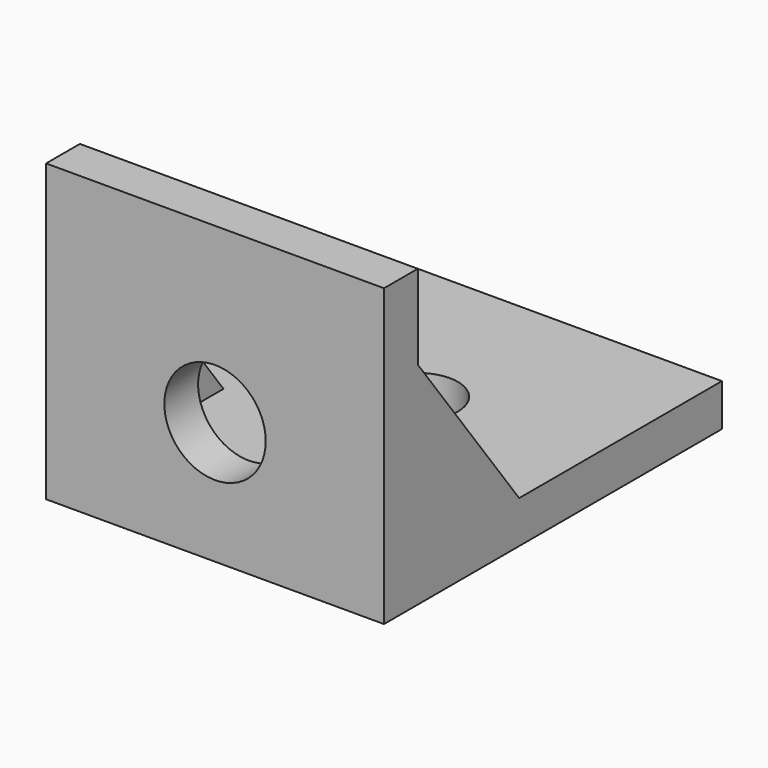
from build123d import *

# Parameters (mm, degrees)
F0_W       = 20
F0_H       = 25
F0_R       = 2.375
F1_DEPTH   = 2.5
F3_DEPTH   = 10
F4_SIZE2   = 7.49999
F4_SIZE    = 9.99999
F4_2_SIZE2 = 7.49999
F4_2_SIZE  = 9.99999
F5_DEPTH   = 5
F6_R       = 3
F7_DEPTH   = 2.5


# Not quite as in the source:
# - a fillet or chamfer is up to 0.001 mm smaller than in the source, because OpenCascade refuses the exact size


with BuildPart() as f1:
    # F0 (on Top) → F1 (new body)
    with BuildSketch(Plane.XY):
        with Locations((-35.0395915519, -25.5869545043)):
            Rectangle(F0_W, F0_H)
        with Locations((-35.0395915519, -23.0869545043)):
            Circle(F0_R, mode=Mode.SUBTRACT)
    extrude(amount=F1_DEPTH)

    # F2 (on face) → F3 (join)
    with BuildSketch(Plane.XY.offset(2.5)):
        Polygon((-42.5395915519, -28.0869545043), (-45.0395915519, -28.0869545043), (-45.0395915519, -38.0869545043), (-25.0395915519, -38.0869545043), (-25.0395915519, -28.0869545043), (-27.5395915519, -28.0869545043), (-27.5395915519, -35.5869545043), (-42.5395915519, -35.5869545043), align=None)
    extrude(amount=F3_DEPTH)

    # F4 (size 10 and 7.5 in the source; OpenCascade refuses exactly that, so slightly less here)
    f4_edges = [f1.edges().sort_by_distance(p)[0] for p in [
        (-43.789592, -28.086955, 12.5),
    ]]
    f4_side = f1.faces().sort_by_distance((-43.789592, -28.086955, 7.5))[0]
    chamfer(f4_edges, length=F4_SIZE, length2=F4_SIZE2, reference=f4_side)

    # F4#2 (size 10 and 7.5 in the source; OpenCascade refuses exactly that, so slightly less here)
    f4_2_edges = [f1.edges().sort_by_distance(p)[0] for p in [
        (-26.289592, -28.086955, 12.5),
    ]]
    f4_2_side = f1.faces().sort_by_distance((-26.289592, -28.086955, 7.5))[0]
    chamfer(f4_2_edges, length=F4_2_SIZE, length2=F4_2_SIZE2, reference=f4_2_side)

    # F5 (add): a face of the model
    f5_faces = [f1.faces().sort_by_distance(p)[0] for p in [
        (-35.0395915519, -36.8369532542, 12.5),
    ]]
    extrude(f5_faces, amount=F5_DEPTH)

    # F6 (on face) → F7 (cut)
    with BuildSketch(Plane.XZ.offset(38.0869545043)):
        with Locations((-35.0395915519, 7.25)):
            Circle(F6_R)
    extrude(amount=-F7_DEPTH, mode=Mode.SUBTRACT)


solid = f1.part
